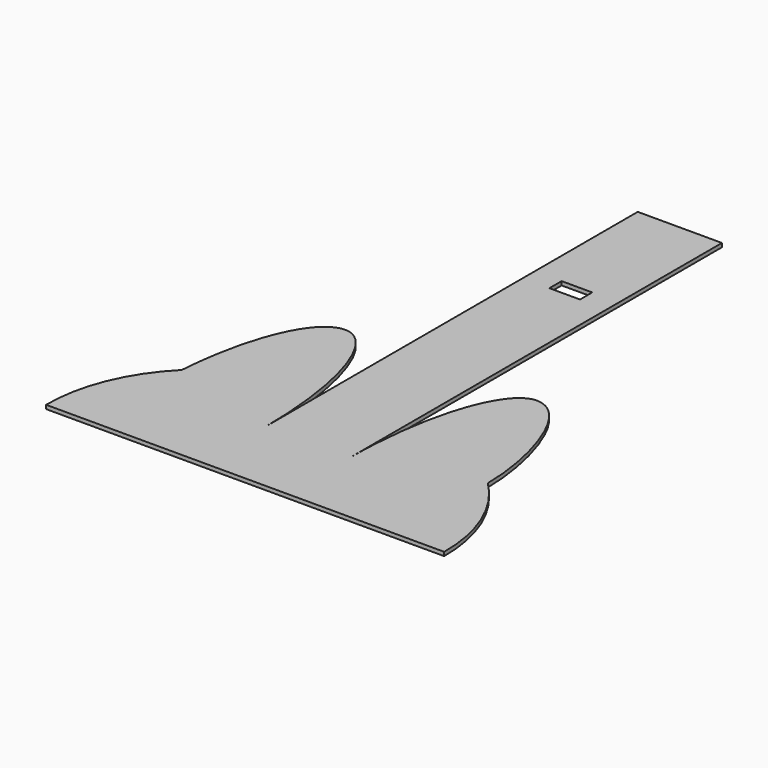
from build123d import *

# Parameters (mm, degrees)
F0_W     = 69.85
F0_H     = 386.08
F0_W_2   = 25.4
F0_H_2   = 12.7
F0_H_3   = 64.6534590532
F1_DEPTH = 3.175


# Not quite as in the source:
# - the dataset's text gives a spline's control points without its knots; the knots are read off the source's solid


with BuildPart() as f1:
    # F0 (on Top) → F1 (new body)
    with BuildSketch(Plane.XY):
        with Locations((34.925, 257.6934590532)):
            Rectangle(F0_W, F0_H)
        with Locations((34.925, 337.7034590532)):
            Rectangle(F0_W_2, F0_H_2, mode=Mode.SUBTRACT)
        with BuildLine():
            Line((0, 0), (0, 64.6534590532))
            add(Edge.make_bspline(
                [(0, 64.6534590532), (0, 203.2), (-44.45, 203.2)],
                knots=[4.7123889804, 4.7123889804, 4.7123889804, 6.2831853072, 6.2831853072, 6.2831853072], degree=2, weights=[1, 0.7071067812, 1]))
            add(Edge.make_bspline(
                [(-44.45, 203.2), (-83.9884760445, 203.2), (-92.075, 92.9894)],
                knots=[0, 0, 0, 1.3648200427, 1.3648200427, 1.3648200427], degree=2, weights=[1, 0.7760550574, 1]))
            ThreePointArc((-92.075, 92.9894), (-120.4661612059, 50.3219990464), (-130.175, 0))
            Line((-130.175, 0), (0, 0))
        make_face()
        with Locations((34.925, 32.3267295266)):
            Rectangle(F0_W, F0_H_3)
        with BuildLine():
            add(Edge.make_bspline(
                [(114.3, 203.2), (116.5605862503, 203.2), (121.9530728583, 202.3331388879), (130.4947147155, 197.5987791483), (141.4933741705, 183.4269013443), (152.7385562531, 156.2534255189), (158.9074917941, 129.7692462355), (161.3044412153, 110.6229696373), (161.8811367628, 98.626656943), (161.925, 92.9830765781)],
                knots=[0.5267526841, 0.5267526841, 0.5267526841, 0.5267526841, 0.5267526841, 0.5267526841, 0.6, 0.7, 0.8, 0.9, 0.9934494331, 0.9934494331, 0.9934494331, 0.9934494331, 0.9934494331, 0.9934494331], degree=5))
            add(Edge.make_bspline(
                [(114.3, 203.2), (69.85, 203.2), (69.85, 64.6534590532)],
                knots=[0, 0, 0, 1.5707963268, 1.5707963268, 1.5707963268], degree=2, weights=[1, 0.7071067812, 1]))
            Line((69.85, 64.6534590532), (69.85, 0))
            Line((69.85, 0), (200.025, 0))
            ThreePointArc((200.025, 0), (190.3149490033, 50.3186009129), (161.925, 92.9830765781))
        make_face()
    extrude(amount=F1_DEPTH)


solid = f1.part
